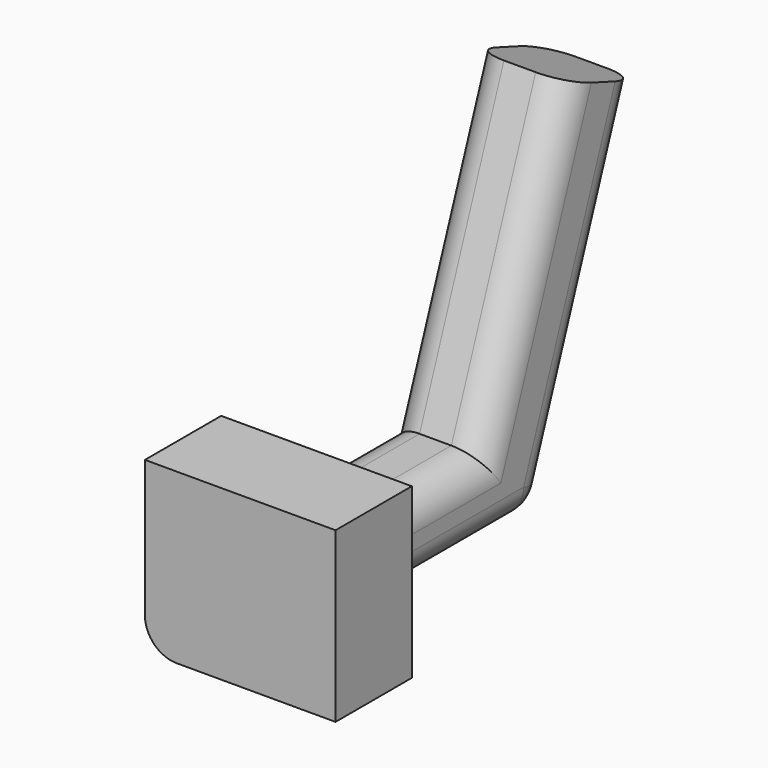
from build123d import *

# Parameters (mm, degrees)
F1_DEPTH     = 6
F2_DEPTH     = 3
F3_R         = 1
F4_R         = 1
F5_R         = 1
F6_R         = 1
F7_R         = 1
F8_R         = 1
F9_T1_DEPTH  = 8.1490483801
F9_T3_DEPTH  = 13.6490483801
F9_T5_DEPTH  = 1
F9_T10_DEPTH = 1
F9_T16_DEPTH = 1


# Not quite as in the source:
# - a fillet or chamfer that OpenCascade refuses, or shapes differently, is made with other operations: its cross-section is extruded or revolved along the edge and cut away or added


with BuildPart() as f1:
    # F0 (on Right) → F1 (new body)
    with BuildSketch(Plane.YZ):
        Polygon((-15.6169078008, 5.0744746653), (-15.6169078008, 7.5457364384), (-15.6169078008, 10.3862823428), (-18.6169078008, 10.3862823428), (-18.6169078008, 5.0744746653), align=None)
    extrude(amount=F1_DEPTH)

    # F0 (on Right) → F2 (join)
    with BuildSketch(Plane.YZ):
        Polygon((-15.6169078008, 5.0744746653), (-15.6169078008, 7.5457364384), (-15.6169078008, 10.3862823428), (-18.6169078008, 10.3862823428), (-18.6169078008, 5.0744746653), align=None)
        Polygon((-9.0572322022, 7.5457364384), (-15.6169078008, 7.5457364384), (-15.6169078008, 5.0744746653), (-6.7705721449, 5.0744746653), (-2.9264162166, 15.5086156212), (-5.7414456778, 16.545731397), align=None)
    extrude(amount=F2_DEPTH)

    # F3
    f3_edges = [f1.edges().sort_by_distance(p)[0] for p in [
        (3, -4.848494, 10.291545),
    ]]
    fillet(f3_edges, radius=F3_R)

    # F4
    f4_edges = [f1.edges().sort_by_distance(p)[0] for p in [
        (3, -7.399339, 12.045734),
    ]]
    fillet(f4_edges, radius=F4_R)

    # F5
    f5_edges = [f1.edges().sort_by_distance(p)[0] for p in [
        (0, -7.399339, 12.045734),
    ]]
    fillet(f5_edges, radius=F5_R)

    # F6
    f6_edges = [f1.edges().sort_by_distance(p)[0] for p in [
        (0, -4.848494, 10.291545),
    ]]
    fillet(f6_edges, radius=F6_R)

    # F7
    f7_edges = [f1.edges().sort_by_distance(p)[0] for p in [
        (3, -12.33707, 7.545736),
    ]]
    fillet(f7_edges, radius=F7_R)

    # F8
    f8_edges = [f1.edges().sort_by_distance(p)[0] for p in [
        (0, -12.33707, 7.545736),
    ]]
    fillet(f8_edges, radius=F8_R)

    # F9: fillet of radius 1 on 3 edges, made by hand

    # F9_s2 → F9_t1 (cut)
    with BuildSketch(Plane.XZ.offset(7.4678594207)):
        with BuildLine():
            ThreePointArc((3, 6.0744746653), (2.7071067812, 5.3673678841), (2, 5.0744746653))
            Line((2, 5.0744746653), (3, 5.0744746653))
            Line((3, 5.0744746653), (3, 6.0744746653))
        make_face()
    extrude(amount=F9_T1_DEPTH, mode=Mode.SUBTRACT)

    # F9_s4 → F9_t3 (cut)
    with BuildSketch(Plane.XZ.offset(7.4678594207)):
        with BuildLine():
            ThreePointArc((0, 6.0744746653), (0.2928932188, 5.3673678841), (1, 5.0744746653))
            Line((1, 5.0744746653), (0, 5.0744746653))
            Line((0, 5.0744746653), (0, 6.0744746653))
        make_face()
    extrude(amount=F9_T3_DEPTH, mode=Mode.SUBTRACT)

    # F9_s6 → F9_t5 (cut)
    with BuildSketch(Plane.YZ.offset(1)):
        with BuildLine():
            ThreePointArc((-7.4678594207, 5.0744746653), (-6.8958914402, 5.2541987182), (-6.5295162669, 5.7287694067))
            Line((-6.5295162669, 5.7287694067), (-6.7705721449, 5.0744746653))
            Line((-6.7705721449, 5.0744746653), (-7.4678594207, 5.0744746653))
        make_face()
    extrude(amount=F9_T5_DEPTH, mode=Mode.SUBTRACT)


with BuildPart() as f9_tool8:
    # F9_s9 → F9_t10 (new body)
    with BuildSketch(Plane.YZ.offset(1)):
        Polygon((-7.4678594207, 6.0744746653), (-7.4678594207, 5.0744746653), (-6.7705721449, 5.0744746653), (-6.5295162669, 5.7287694067), align=None)
    extrude(amount=-F9_T10_DEPTH)

    # F9_s11 → F9_t12 (revolve, cut)
    with BuildSketch(Plane(origin=(1, -7.4678594207, 6.0744746653), x_dir=(0, -0.5719679805, 0.820275947), z_dir=(0, -0.820275947, -0.5719679805))):
        with BuildLine():
            ThreePointArc((0, -1), (1, 0), (0, 1))
            Line((0, 1), (0, -1))
        make_face()
    revolve(axis=Axis((1, -7.4678594207, 6.0744746653), (-1, 0, 0)), mode=Mode.SUBTRACT)


with BuildPart() as f1_1:
    add(f1.part)

    # F9_t7: cut F9_tool8
    add(f9_tool8.part, mode=Mode.SUBTRACT)


with BuildPart() as f9_tool14:
    # F9_s15 → F9_t16 (new body)
    with BuildSketch(Plane.YZ.offset(2)):
        Polygon((-7.4678594207, 6.0744746653), (-7.4678594207, 5.0744746653), (-6.7705721449, 5.0744746653), (-6.5295162669, 5.7287694067), align=None)
    extrude(amount=F9_T16_DEPTH)

    # F9_s17 → F9_t18 (revolve, cut)
    with BuildSketch(Plane(origin=(2, -7.4678594207, 6.0744746653), x_dir=(0, -0.5719679805, 0.820275947), z_dir=(0, 0.820275947, 0.5719679805))):
        with BuildLine():
            ThreePointArc((0, -1), (1, 0), (0, 1))
            Line((0, 1), (0, -1))
        make_face()
    revolve(axis=Axis((2, -7.4678594207, 6.0744746653), (1, 0, 0)), mode=Mode.SUBTRACT)


with BuildPart() as f1_2:
    add(f1_1.part)

    # F9_t13: cut F9_tool14
    add(f9_tool14.part, mode=Mode.SUBTRACT)


solid = f1_2.part
